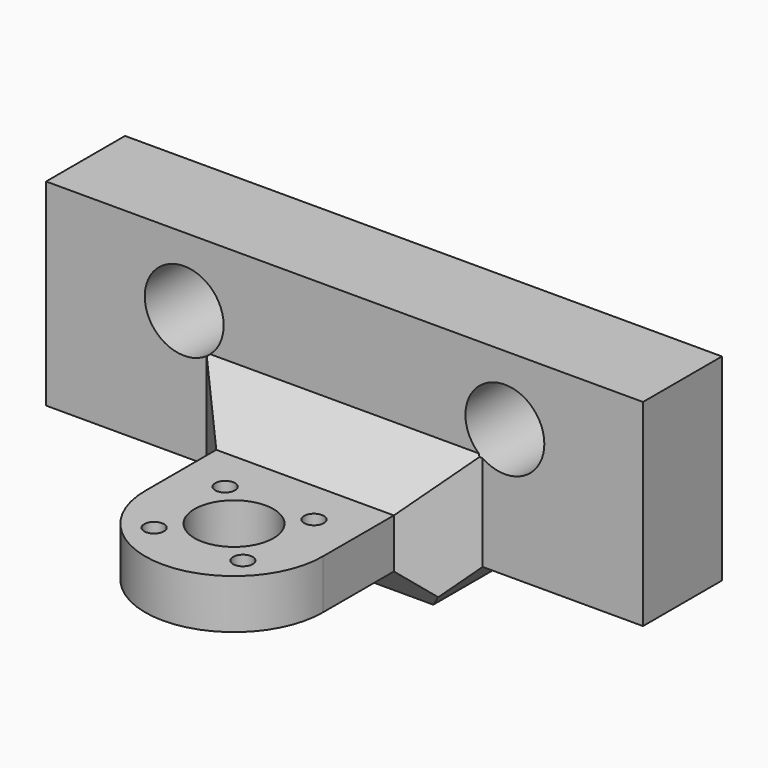
from build123d import *

# Parameters (mm, degrees)
F0_R         = 1
F0_W         = 18
F0_H         = 10
F1_DEPTH     = 5
F0_W_2       = 21.25
F0_R_2       = 4
F2_DEPTH     = 20
F3_R         = 4
F4_DEPTH     = 25
F5_DEPTH     = 5
F6_T4_DEPTH  = 18
F7_T1_DEPTH  = 5
F7_T3_DEPTH  = 18
F7_T8_DEPTH  = 10
F7_T13_DEPTH = 10
F7_T19_DEPTH = 22.8584149398
F7_T24_DEPTH = 17.8584149398
F7_T33_DEPTH = 30.8584149398
F7_S35_R     = 4
F7_T36_DEPTH = 17
F7_T39_DEPTH = 17.8584149398
F7_S41_R     = 4
F7_T42_DEPTH = 11
F7_T48_DEPTH = 30.8584149398
F7_S50_R     = 4
F7_T51_DEPTH = 17
F7_T54_DEPTH = 17.8584149398
F7_S56_R     = 4
F7_T57_DEPTH = 11
F7_T63_DEPTH = 17.8584149398
F7_T69_DEPTH = 22.8584149398


# Not quite as in the source:
# - a fillet or chamfer that OpenCascade refuses, or shapes differently, is made with other operations: its cross-section is extruded or revolved along the edge and cut away or added
# - a feature names something its author has since deleted; it is built from what else it names


with BuildPart() as f1:
    # F0 (on Top) → F1 (new body)
    with BuildSketch(Plane.XY):
        with BuildLine():
            Line((9, 0), (4, 0))
            ThreePointArc((4, 0), (0, -4), (-4, 0))
            Line((-4, 0), (-9, 0))
            ThreePointArc((-9, 0), (0, -9), (9, 0))
        make_face()
        with Locations((-4.5, -4.5)):
            Circle(F0_R, mode=Mode.SUBTRACT)
        with Locations((4.5, -4.5)):
            Circle(F0_R, mode=Mode.SUBTRACT)
        with BuildLine():
            ThreePointArc((-4, 0), (0, 4), (4, 0))
            Line((4, 0), (9, 0))
            ThreePointArc((9, 0), (0, 9), (-9, 0))
            Line((-9, 0), (-4, 0))
        make_face()
        with BuildLine():
            ThreePointArc((-4.5, 3.5), (-5.2071067812, 5.2071067812), (-3.5, 4.5))
            ThreePointArc((-3.5, 4.5), (-3.7928932188, 3.7928932188), (-4.5, 3.5))
        make_face(mode=Mode.SUBTRACT)
        with Locations((4.5, 4.5)):
            Circle(F0_R, mode=Mode.SUBTRACT)
        with BuildLine():
            ThreePointArc((-9, 0), (0, 9), (9, 0))
            Line((9, 0), (9, 14))
            Line((9, 14), (-9, 14))
            Line((-9, 14), (-9, 0))
        make_face()
        with Locations((0, 19)):
            Rectangle(F0_W, F0_H)
    extrude(amount=F1_DEPTH)

    # F0 (on Top) → F2 (join)
    with BuildSketch(Plane.XY):
        with Locations((0, 19)):
            Rectangle(F0_W, F0_H)
        with Locations((-19.625, 19)):
            Rectangle(F0_W_2, F0_H)
        with Locations((-20.25, 19)):
            Circle(F0_R_2, mode=Mode.SUBTRACT)
        with Locations((19.625, 19)):
            Rectangle(F0_W_2, F0_H)
        with Locations((20.25, 19)):
            Circle(F0_R_2, mode=Mode.SUBTRACT)
        with Locations((20.25, 19)):
            Circle(F0_R_2)
        with Locations((-20.25, 19)):
            Circle(F0_R_2)
    extrude(amount=F2_DEPTH)

    # F3 (on Front) → F4 (cut)
    with BuildSketch(Plane.XZ):
        with Locations((-16.25, 13)):
            Circle(F3_R)
        with Locations((16.25, 13)):
            Circle(F3_R)
    extrude(amount=-F4_DEPTH, mode=Mode.SUBTRACT)

    # F0 (on Top) → F5 (join)
    with BuildSketch(Plane.XY):
        with Locations((0, 19)):
            Rectangle(F0_W, F0_H)
    extrude(amount=-F5_DEPTH)

    # F6: chamfer of 5 on 1 edges, made by hand


with BuildPart() as f6_tool2:
    # F6_s3 → F6_t4 (new body)
    with BuildSketch(Plane.YZ.offset(-9)):
        Polygon((9, 0), (14, -5), (14, 0), align=None)
    extrude(amount=F6_T4_DEPTH)

    split(bisect_by=Plane.XY.offset(-5), keep=Keep.TOP)


with BuildPart() as f1_1:
    add(f1.part)

    # F6_t1: union F6_tool2
    add(f6_tool2.part)

    # F7: chamfer of 5 on 5 edges, made by hand

    # F7_s2 → F7_t1 (join)
    with BuildSketch(Plane.XY):
        Polygon((-9, 9), (-14, 14), (-9, 14), align=None)
        Polygon((9, 9), (14, 14), (9, 14), align=None)
    extrude(amount=F7_T1_DEPTH)

    # F7_s4 → F7_t3 (join)
    with BuildSketch(Plane.YZ.offset(-9)):
        Polygon((9, 5), (14, 10), (14, 5), align=None)
    extrude(amount=F7_T3_DEPTH)


with BuildPart() as f7_tool6:
    # F7_s7 → F7_t8 (new body)
    with BuildSketch(Plane.XZ.offset(-14)):
        Polygon((9, -5), (14, 0), (9, 0), align=None)
    extrude(amount=-F7_T8_DEPTH)

    split(bisect_by=Plane.XY.offset(-5), keep=Keep.TOP)


with BuildPart() as f1_2:
    add(f1_1.part)

    # F7_t5: union F7_tool6
    add(f7_tool6.part)


with BuildPart() as f7_tool11:
    # F7_s12 → F7_t13 (new body)
    with BuildSketch(Plane.XZ.offset(-24)):
        Polygon((-9, -5), (-14, 0), (-9, 0), align=None)
    extrude(amount=F7_T13_DEPTH)

    split(bisect_by=Plane.XY.offset(-5), keep=Keep.TOP)


with BuildPart() as f1_3:
    add(f1_2.part)

    # F7_t10: union F7_tool11
    add(f7_tool11.part)


with BuildPart() as f7_tool17:
    # F7_s18 → F7_t19 (new body)
    with BuildSketch(Plane.XZ.offset(-24)):
        Polygon((-9, -5), (-14, 0), (-9, 0), align=None)
    extrude(amount=F7_T19_DEPTH)

    split(bisect_by=Plane(origin=(0, 4.5, 4.5), x_dir=(1, 0, 0), z_dir=(0, 0.7071067812, 0.7071067812)), keep=Keep.TOP)

    split(bisect_by=Plane.XZ.offset(-14), keep=Keep.TOP)


with BuildPart() as f7_tool22:
    # F7_s23 → F7_t24 (new body)
    with BuildSketch(Plane.XY.offset(-12.8584149398)):
        Polygon((-9, 9), (-14, 14), (-9, 14), align=None)
    extrude(amount=F7_T24_DEPTH)

    split(bisect_by=Plane.XY, keep=Keep.BOTTOM)

    split(bisect_by=Plane(origin=(0, 4.5, 4.5), x_dir=(1, 0, 0), z_dir=(0, 0.7071067812, 0.7071067812)), keep=Keep.TOP)

    split(bisect_by=Plane.XY.offset(-5), keep=Keep.TOP)


with BuildPart() as f7_tool17_1:
    add(f7_tool17.part)

    # F7_t28: intersect F7_tool22
    add(f7_tool22.part, mode=Mode.INTERSECT)


with BuildPart() as f1_4:
    add(f1_3.part)

    # F7_t15: union F7_tool17
    add(f7_tool17_1.part)


with BuildPart() as f7_tool31:
    # F7_s32 → F7_t33 (new body)
    with BuildSketch(Plane.YZ.offset(9)):
        Polygon((9, 5), (14, 10), (14, 5), align=None)
    extrude(amount=-F7_T33_DEPTH)

    split(bisect_by=Plane.YZ.offset(-9), keep=Keep.BOTTOM)

    # F7_s35 → F7_t36 (cut, symmetric)
    with BuildSketch(Plane.XZ.offset(-11.5)):
        with Locations((-16.25, 13)):
            Circle(F7_S35_R)
    extrude(amount=F7_T36_DEPTH, both=True, mode=Mode.SUBTRACT)


with BuildPart() as f7_tool37:
    # F7_s38 → F7_t39 (new body)
    with BuildSketch(Plane.XY):
        Polygon((-9, 9), (-14, 14), (-9, 14), align=None)
    extrude(amount=F7_T39_DEPTH)

    split(bisect_by=Plane.XY.offset(5), keep=Keep.TOP)

    # F7_s41 → F7_t42 (cut, symmetric)
    with BuildSketch(Plane.XZ.offset(-11.5)):
        with Locations((-16.25, 13)):
            Circle(F7_S41_R)
    extrude(amount=F7_T42_DEPTH, both=True, mode=Mode.SUBTRACT)


with BuildPart() as f7_tool31_1:
    add(f7_tool31.part)

    # F7_t43: intersect F7_tool37
    add(f7_tool37.part, mode=Mode.INTERSECT)


with BuildPart() as f1_5:
    add(f1_4.part)

    # F7_t29: union F7_tool31
    add(f7_tool31_1.part)


with BuildPart() as f7_tool46:
    # F7_s47 → F7_t48 (new body)
    with BuildSketch(Plane.YZ.offset(21.8584149398)):
        Polygon((9, 5), (14, 10), (14, 5), align=None)
    extrude(amount=-F7_T48_DEPTH)

    split(bisect_by=Plane.YZ.offset(9), keep=Keep.TOP)

    # F7_s50 → F7_t51 (cut, symmetric)
    with BuildSketch(Plane.XZ.offset(-11.5)):
        with Locations((16.25, 13)):
            Circle(F7_S50_R)
    extrude(amount=F7_T51_DEPTH, both=True, mode=Mode.SUBTRACT)


with BuildPart() as f7_tool52:
    # F7_s53 → F7_t54 (new body)
    with BuildSketch(Plane.XY.offset(17.8584149398)):
        Polygon((9, 9), (14, 14), (9, 14), align=None)
    extrude(amount=-F7_T54_DEPTH)

    split(bisect_by=Plane.XY.offset(5), keep=Keep.TOP)

    # F7_s56 → F7_t57 (cut, symmetric)
    with BuildSketch(Plane.XZ.offset(-11.5)):
        with Locations((16.25, 13)):
            Circle(F7_S56_R)
    extrude(amount=F7_T57_DEPTH, both=True, mode=Mode.SUBTRACT)


with BuildPart() as f7_tool46_1:
    add(f7_tool46.part)

    # F7_t58: intersect F7_tool52
    add(f7_tool52.part, mode=Mode.INTERSECT)


with BuildPart() as f1_6:
    add(f1_5.part)

    # F7_t44: union F7_tool46
    add(f7_tool46_1.part)


with BuildPart() as f7_tool61:
    # F7_s62 → F7_t63 (new body)
    with BuildSketch(Plane.XY.offset(5)):
        Polygon((9, 9), (14, 14), (9, 14), align=None)
    extrude(amount=-F7_T63_DEPTH)

    split(bisect_by=Plane.XY, keep=Keep.BOTTOM)

    split(bisect_by=Plane(origin=(0, 4.5, 4.5), x_dir=(1, 0, 0), z_dir=(0, 0.7071067812, 0.7071067812)), keep=Keep.TOP)

    split(bisect_by=Plane.XY.offset(-5), keep=Keep.TOP)


with BuildPart() as f7_tool67:
    # F7_s68 → F7_t69 (new body)
    with BuildSketch(Plane.XZ.offset(-1.1415850602)):
        Polygon((9, -5), (14, 0), (9, 0), align=None)
    extrude(amount=-F7_T69_DEPTH)

    split(bisect_by=Plane(origin=(0, 4.5, 4.5), x_dir=(1, 0, 0), z_dir=(0, 0.7071067812, 0.7071067812)), keep=Keep.TOP)

    split(bisect_by=Plane.XZ.offset(-14), keep=Keep.TOP)


with BuildPart() as f7_tool61_1:
    add(f7_tool61.part)

    # F7_t72: intersect F7_tool67
    add(f7_tool67.part, mode=Mode.INTERSECT)


with BuildPart() as f1_7:
    add(f1_6.part)

    # F7_t59: union F7_tool61
    add(f7_tool61_1.part)


solid = f1_7.part
